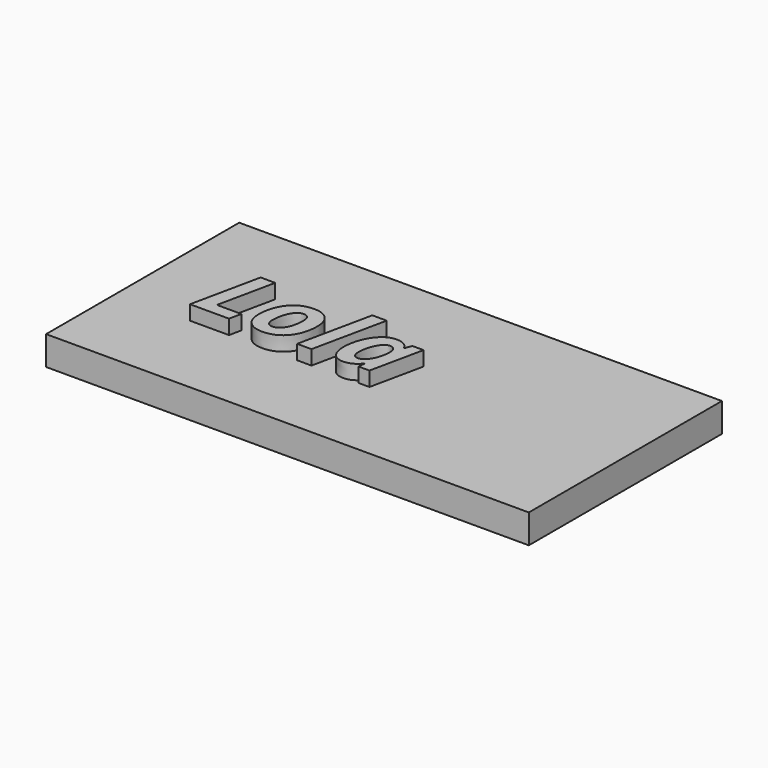
from build123d import *

# Parameters (mm, degrees)
F0_W         = 100
F0_H         = 50
F1_DEPTH     = 3
F2_DEPTH     = 3
F3_TEXT_SIZE = 20.2609846989
F4_DEPTH     = 3


# Not quite as in the source:
# - a feature names something its author has since deleted; it is built from what else it names
# - Text() gives the source's letters only with a copy of the font that has no kerning and outlines rounded to 1/6400 em; it was checked with that copy


with BuildPart() as f1:
    # F0 (on Top) → F1 (new body)
    with BuildSketch(Plane.XY):
        with Locations((-50, 25)):
            Rectangle(F0_W, F0_H)
    extrude(amount=F1_DEPTH)

    # F2 (add): a face of the model
    f2_faces = [f1.faces().sort_by_distance(p)[0] for p in [
        (-50, 25, 3),
    ]]
    extrude(f2_faces, amount=F2_DEPTH)

    # F3 (on face) → F4 (join)
    with BuildSketch(Plane.XY.offset(6)):
        with Locations((-85.2854400873, 18.2107500732)):
            Text('Lola', F3_TEXT_SIZE, font='Open Sans', font_style=FontStyle.BOLDITALIC, text_align=(TextAlign.LEFT, TextAlign.BOTTOM))
    extrude(amount=F4_DEPTH)


solid = f1.part
